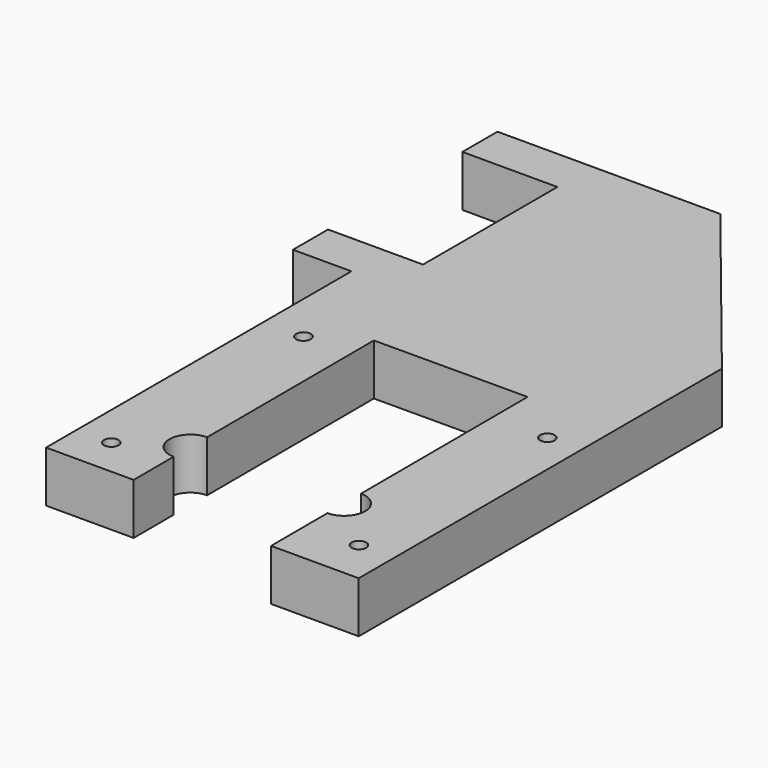
from build123d import *

# Parameters (mm, degrees)
F1_DEPTH = 7
F2_D     = 2
F3_D     = 5.75
F4_DEPTH = 16
F5_DEPTH = 5


with BuildPart() as f1:
    # F0 (on Top) → F1 (new body)
    with BuildSketch(Plane.XY):
        Polygon((10.5, -45), (22.5, -45), (22.5, 17.153987661), (0, 45), (-14.5, 45), (-14.5, 39), (-22.5, 39), (-22.5, 16), (-14.5, 16), (-14.5, 10), (-22.5, 10), (-22.5, -42.25), (-10.5080957781, -42.25), (-10.6281967604, -1.0001864958), (10.3717142302, -0.9390441602), align=None)
    extrude(amount=F1_DEPTH)

    # F2 (through all)
    with Locations(Plane(origin=(0, 0, 0), x_dir=(1, 0, 0), z_dir=(0, 0, -1))):
        with Locations((-17.0669870824, 5), (-17.7734121563, 37), (17.7265878437, 39), (17.9330129176, 7)):
            Hole(F2_D / 2)

    # F3 (through all)
    with Locations(Plane(origin=(0, 0, 0), x_dir=(1, 0, 0), z_dir=(0, 0, -1))):
        with Locations((-10.5364832571, 32.5000529818), (10.4634277335, 32.4389106462)):
            Hole(F3_D / 2)

    # F4 (add): faces of the model
    f4_faces = [f1.faces().sort_by_distance(p)[0] for p in [
        (-14.5, 42, 3.5),
        (-14.5, 13, 3.5),
    ]]
    extrude(f4_faces, amount=F4_DEPTH)

    # F5 (cut): a face of the model
    f5_faces = [f1.faces().sort_by_distance(p)[0] for p in [
        (-22.5, 27.5, 3.5),
    ]]
    extrude(f5_faces, amount=-F5_DEPTH, mode=Mode.SUBTRACT)


solid = f1.part
